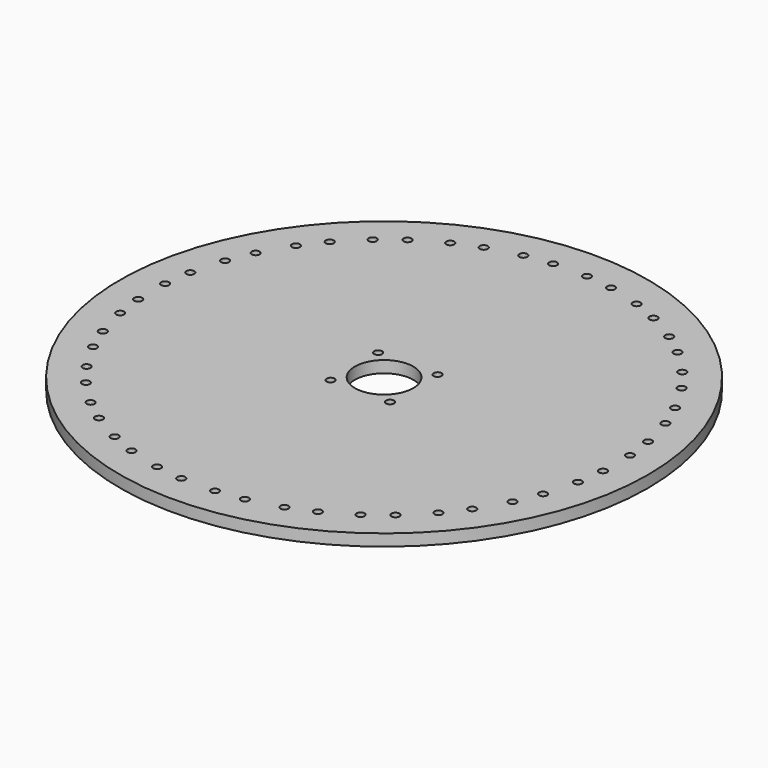
from build123d import *

# Parameters (mm, degrees)
F0_R            = 114.6499739
F0_R_2          = 1.7272
F0_R_3          = 12.7
F1_DEPTH        = 5.08
F2_R            = 1.7272
F3_DEPTH        = 5.08
F3_COPIES_COUNT = 24


# Not quite as in the source:
# - a pattern or mirror of a feature is missing from the dataset's text; its kind, count and spacing are read off the source's solid


with BuildPart() as f1:
    # F0 (on Top) → F1 (new body)
    with BuildSketch(Plane.XY):
        Circle(F0_R)
        with Locations((-12.909118174, -12.909118174)):
            Circle(F0_R_2, mode=Mode.SUBTRACT)
        with Locations((12.909118174, -12.909118174)):
            Circle(F0_R_2, mode=Mode.SUBTRACT)
        with Locations((-12.909118174, 12.909118174)):
            Circle(F0_R_2, mode=Mode.SUBTRACT)
        Circle(F0_R_3, mode=Mode.SUBTRACT)
        with Locations((12.909118174, 12.909118174)):
            Circle(F0_R_2, mode=Mode.SUBTRACT)
    extrude(amount=F1_DEPTH)

    # F2 (on face) → F3 (cut, through all)
    with BuildSketch(Plane.XY.offset(5.08)):
        with Locations((19.05, -99.4099739)):
            Circle(F2_R)
        with Locations((-19.05, -99.4099739)):
            Circle(F2_R)
    f3 = extrude(amount=-F3_DEPTH, mode=Mode.SUBTRACT)

    # F3_copies: F3 ×24 about axis
    f3_copies_axis = Axis((0, 0, 0), (0, 0, 1))
    for i in range(1, F3_COPIES_COUNT):
        add(f3.rotate(f3_copies_axis, i * 360 / F3_COPIES_COUNT), mode=Mode.SUBTRACT)


solid = f1.part
